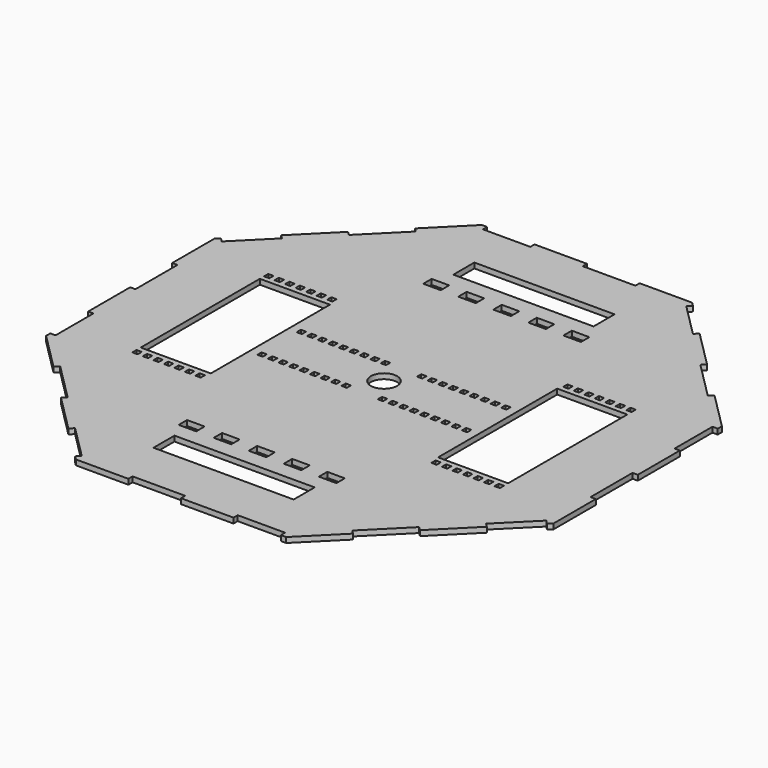
from build123d import *

# Parameters (mm, degrees)
F0_W     = 10
F0_H     = 6
F0_W_2   = 3
F0_H_2   = 2.9955762632
F0_H_3   = 3
F0_H_4   = 3.0048715621
F0_W_3   = 80
F0_H_5   = 15
F0_R     = 7.5
F1_DEPTH = 1.5


with BuildPart() as f1:
    # F0 (on Top) → F1 (new body, symmetric)
    with BuildSketch(Plane.XY):
        Polygon((-57, 144.85), (-59.9988345097, 144.85), (-81.2120379453, 123.6367965644), (-79.0907176018, 121.5154762208), (-100.3039210374, 100.3022727852), (-102.4252413776, 102.4235931255), (-123.6384448165, 81.2103896932), (-121.5171244733, 79.0890693493), (-140.6090075683, 59.9971862603), (-142.7303279089, 62.1185066008), (-144.85, 59.9988345097), (-144.85, 29.9988345097), (-141.85, 29.9988345097), (-141.85, -0.0011654903), (-144.85, 0), (-144.85, -30), (-141.85, -30), (-141.85, -57), (-144.85, -57), (-144.85, -59.9988345097), (-123.6367965644, -81.2120379453), (-121.5154762208, -79.0907176018), (-100.3022727852, -100.3039210374), (-102.4235931255, -102.4252413776), (-81.2103896932, -123.6384448165), (-79.0890693493, -121.5171244733), (-59.9971862603, -140.6090075683), (-62.1185066012, -142.7303279086), (-59.9988345097, -144.85), (-29.9988345097, -144.85), (-29.9988345097, -141.85), (0, -141.85), (0, -144.85), (30, -144.85), (30, -141.85), (56.9988345097, -141.85), (56.9988345097, -144.85), (59.9988345097, -144.85), (81.2120379453, -123.6367965644), (79.0907176018, -121.5154762208), (100.3039210374, -100.3022727852), (102.4252413809, -102.4235931288), (123.6384448165, -81.2103896932), (121.517124473, -79.0890693497), (140.609007565, -59.9971862576), (142.7303279086, -62.1185066012), (144.85, -59.9988345097), (144.85, -29.9988345097), (141.85, -29.9988345097), (141.85, 0.0011654903), (144.85, 0), (144.85, 30), (141.85, 30), (141.85, 57), (144.85, 57), (144.85, 59.9988345097), (123.6367965644, 81.2120379453), (121.5154762208, 79.0907176018), (100.3022727852, 100.3039210374), (102.4235931255, 102.4252413776), (81.2103896932, 123.6384448165), (79.0890693497, 121.517124473), (59.9971862576, 140.609007565), (62.1185066012, 142.7303279086), (59.9988345097, 144.85), (29.9988345097, 144.85), (29.9988345097, 141.85), (-0.0011654903, 141.85), (0, 144.85), (-30, 144.85), (-30, 141.85), (-57, 141.85), align=None)
        with Locations((-40, -87.228587389)):
            Rectangle(F0_W, F0_H, mode=Mode.SUBTRACT)
        with Locations((-20, -87.228587389)):
            Rectangle(F0_W, F0_H, mode=Mode.SUBTRACT)
        with Locations((-103.35, -46.9933643948)):
            Rectangle(F0_W_2, F0_H_2, mode=Mode.SUBTRACT)
        with Locations((-97.35, -46.9911525264)):
            Rectangle(F0_W_2, F0_H_3, mode=Mode.SUBTRACT)
        with Locations((-91.3500337635, -46.9911525264)):
            Rectangle(F0_W_2, F0_H_3, mode=Mode.SUBTRACT)
        Polygon((-83.8500467715, -48.4911525264), (-86.8500337635, -48.4911525264), (-86.8500337635, -45.4911525264), (-83.8500337635, -45.4911525264), align=None, mode=Mode.SUBTRACT)
        with Locations((-79.3500130463, -46.9911525264)):
            Rectangle(F0_W_2, F0_H_3, mode=Mode.SUBTRACT)
        with Locations((-73.3500130463, -46.9911525264)):
            Rectangle(F0_W_2, F0_H_3, mode=Mode.SUBTRACT)
        with Locations((-67.3500130463, -46.9911525264)):
            Rectangle(F0_W_2, F0_H_3, mode=Mode.SUBTRACT)
        with Locations((-58.35, -14)):
            Rectangle(F0_W_2, F0_H_3, mode=Mode.SUBTRACT)
        with Locations((-52.35, -14)):
            Rectangle(F0_W_2, F0_H_3, mode=Mode.SUBTRACT)
        with Locations((-46.35, -13.9975642189)):
            Rectangle(F0_W_2, F0_H_4, mode=Mode.SUBTRACT)
        with Locations((-40.35, -14)):
            Rectangle(F0_W_2, F0_H_3, mode=Mode.SUBTRACT)
        with Locations((-34.35, -14)):
            Rectangle(F0_W_2, F0_H_3, mode=Mode.SUBTRACT)
        with Locations((-28.35, -14)):
            Rectangle(F0_W_2, F0_H_3, mode=Mode.SUBTRACT)
        with Locations((-22.35, -14)):
            Rectangle(F0_W_2, F0_H_3, mode=Mode.SUBTRACT)
        with Locations((-16.35, -14)):
            Rectangle(F0_W_2, F0_H_3, mode=Mode.SUBTRACT)
        with Locations((-10.35, -14)):
            Rectangle(F0_W_2, F0_H_3, mode=Mode.SUBTRACT)
        with Locations((0, -106.9599688053)):
            Rectangle(F0_W_3, F0_H_5, mode=Mode.SUBTRACT)
        with Locations((0, -87.228587389)):
            Rectangle(F0_W, F0_H, mode=Mode.SUBTRACT)
        with Locations((20, -87.228587389)):
            Rectangle(F0_W, F0_H, mode=Mode.SUBTRACT)
        with Locations((40, -87.228587389)):
            Rectangle(F0_W, F0_H, mode=Mode.SUBTRACT)
        with Locations((67.3500130463, -46.9911525264)):
            Rectangle(F0_W_2, F0_H_3, mode=Mode.SUBTRACT)
        with Locations((10.35, -14)):
            Rectangle(F0_W_2, F0_H_3, mode=Mode.SUBTRACT)
        with Locations((16.35, -14)):
            Rectangle(F0_W_2, F0_H_3, mode=Mode.SUBTRACT)
        with Locations((22.35, -14)):
            Rectangle(F0_W_2, F0_H_3, mode=Mode.SUBTRACT)
        with Locations((28.35, -14)):
            Rectangle(F0_W_2, F0_H_3, mode=Mode.SUBTRACT)
        with Locations((34.35, -14)):
            Rectangle(F0_W_2, F0_H_3, mode=Mode.SUBTRACT)
        with Locations((40.35, -14)):
            Rectangle(F0_W_2, F0_H_3, mode=Mode.SUBTRACT)
        with Locations((46.35, -13.9975642189)):
            Rectangle(F0_W_2, F0_H_4, mode=Mode.SUBTRACT)
        with Locations((52.35, -14)):
            Rectangle(F0_W_2, F0_H_3, mode=Mode.SUBTRACT)
        with Locations((58.35, -14)):
            Rectangle(F0_W_2, F0_H_3, mode=Mode.SUBTRACT)
        with Locations((73.3500130463, -46.9911525264)):
            Rectangle(F0_W_2, F0_H_3, mode=Mode.SUBTRACT)
        with Locations((79.3500130463, -46.9911525264)):
            Rectangle(F0_W_2, F0_H_3, mode=Mode.SUBTRACT)
        Polygon((86.8500337635, -45.4911525264), (86.8500337635, -48.4911525264), (83.8500467715, -48.4911525264), (83.8500337635, -45.4911525264), align=None, mode=Mode.SUBTRACT)
        with Locations((91.3500337635, -46.9911525264)):
            Rectangle(F0_W_2, F0_H_3, mode=Mode.SUBTRACT)
        with Locations((97.35, -46.9911525264)):
            Rectangle(F0_W_2, F0_H_3, mode=Mode.SUBTRACT)
        with Locations((103.35, -46.9933643948)):
            Rectangle(F0_W_2, F0_H_2, mode=Mode.SUBTRACT)
        Polygon((-104.85, -42.5), (-104.85, 0), (-104.85, 42.5), (-64.85, 42.5), (-64.85, -42.5), align=None, mode=Mode.SUBTRACT)
        with Locations((-103.35, 46.9933643948)):
            Rectangle(F0_W_2, F0_H_2, mode=Mode.SUBTRACT)
        with Locations((-97.35, 46.9911525264)):
            Rectangle(F0_W_2, F0_H_3, mode=Mode.SUBTRACT)
        with Locations((-91.3500337635, 46.9911525264)):
            Rectangle(F0_W_2, F0_H_3, mode=Mode.SUBTRACT)
        Polygon((-86.8500337635, 45.4911525264), (-86.8500337635, 48.4911525264), (-83.8500467715, 48.4911525264), (-83.8500337635, 45.4911525264), align=None, mode=Mode.SUBTRACT)
        with Locations((-79.3500130463, 46.9911525264)):
            Rectangle(F0_W_2, F0_H_3, mode=Mode.SUBTRACT)
        with Locations((-73.3500130463, 46.9911525264)):
            Rectangle(F0_W_2, F0_H_3, mode=Mode.SUBTRACT)
        with Locations((-58.35, 14)):
            Rectangle(F0_W_2, F0_H_3, mode=Mode.SUBTRACT)
        with Locations((-52.35, 14)):
            Rectangle(F0_W_2, F0_H_3, mode=Mode.SUBTRACT)
        with Locations((-46.35, 13.9975642189)):
            Rectangle(F0_W_2, F0_H_4, mode=Mode.SUBTRACT)
        with Locations((-40.35, 14)):
            Rectangle(F0_W_2, F0_H_3, mode=Mode.SUBTRACT)
        with Locations((-34.35, 14)):
            Rectangle(F0_W_2, F0_H_3, mode=Mode.SUBTRACT)
        with Locations((-28.35, 14)):
            Rectangle(F0_W_2, F0_H_3, mode=Mode.SUBTRACT)
        with Locations((-22.35, 14)):
            Rectangle(F0_W_2, F0_H_3, mode=Mode.SUBTRACT)
        with Locations((-16.35, 14)):
            Rectangle(F0_W_2, F0_H_3, mode=Mode.SUBTRACT)
        with Locations((-10.35, 14)):
            Rectangle(F0_W_2, F0_H_3, mode=Mode.SUBTRACT)
        with Locations((-67.3500130463, 46.9911525264)):
            Rectangle(F0_W_2, F0_H_3, mode=Mode.SUBTRACT)
        with Locations((-40, 87.228587389)):
            Rectangle(F0_W, F0_H, mode=Mode.SUBTRACT)
        with Locations((-20, 87.228587389)):
            Rectangle(F0_W, F0_H, mode=Mode.SUBTRACT)
        Circle(F0_R, mode=Mode.SUBTRACT)
        with Locations((10.35, 14)):
            Rectangle(F0_W_2, F0_H_3, mode=Mode.SUBTRACT)
        with Locations((16.35, 14)):
            Rectangle(F0_W_2, F0_H_3, mode=Mode.SUBTRACT)
        with Locations((22.35, 14)):
            Rectangle(F0_W_2, F0_H_3, mode=Mode.SUBTRACT)
        with Locations((28.35, 14)):
            Rectangle(F0_W_2, F0_H_3, mode=Mode.SUBTRACT)
        with Locations((34.35, 14)):
            Rectangle(F0_W_2, F0_H_3, mode=Mode.SUBTRACT)
        with Locations((40.35, 14)):
            Rectangle(F0_W_2, F0_H_3, mode=Mode.SUBTRACT)
        with Locations((46.35, 13.9975642189)):
            Rectangle(F0_W_2, F0_H_4, mode=Mode.SUBTRACT)
        with Locations((52.35, 14)):
            Rectangle(F0_W_2, F0_H_3, mode=Mode.SUBTRACT)
        with Locations((58.35, 14)):
            Rectangle(F0_W_2, F0_H_3, mode=Mode.SUBTRACT)
        with Locations((67.3500130463, 46.9911525264)):
            Rectangle(F0_W_2, F0_H_3, mode=Mode.SUBTRACT)
        Polygon((104.85, 0), (104.85, -42.5), (64.85, -42.5), (64.85, 42.5), (104.85, 42.5), align=None, mode=Mode.SUBTRACT)
        with Locations((73.3500130463, 46.9911525264)):
            Rectangle(F0_W_2, F0_H_3, mode=Mode.SUBTRACT)
        with Locations((79.3500130463, 46.9911525264)):
            Rectangle(F0_W_2, F0_H_3, mode=Mode.SUBTRACT)
        Polygon((83.8500467715, 48.4911525264), (86.8500337635, 48.4911525264), (86.8500337635, 45.4911525264), (83.8500337635, 45.4911525264), align=None, mode=Mode.SUBTRACT)
        with Locations((91.3500337635, 46.9911525264)):
            Rectangle(F0_W_2, F0_H_3, mode=Mode.SUBTRACT)
        with Locations((97.35, 46.9911525264)):
            Rectangle(F0_W_2, F0_H_3, mode=Mode.SUBTRACT)
        with Locations((103.35, 46.9933643948)):
            Rectangle(F0_W_2, F0_H_2, mode=Mode.SUBTRACT)
        with Locations((0, 87.228587389)):
            Rectangle(F0_W, F0_H, mode=Mode.SUBTRACT)
        with Locations((20, 87.228587389)):
            Rectangle(F0_W, F0_H, mode=Mode.SUBTRACT)
        with Locations((0, 106.9599688053)):
            Rectangle(F0_W_3, F0_H_5, mode=Mode.SUBTRACT)
        with Locations((40, 87.228587389)):
            Rectangle(F0_W, F0_H, mode=Mode.SUBTRACT)
    extrude(amount=F1_DEPTH, both=True)


solid = f1.part
